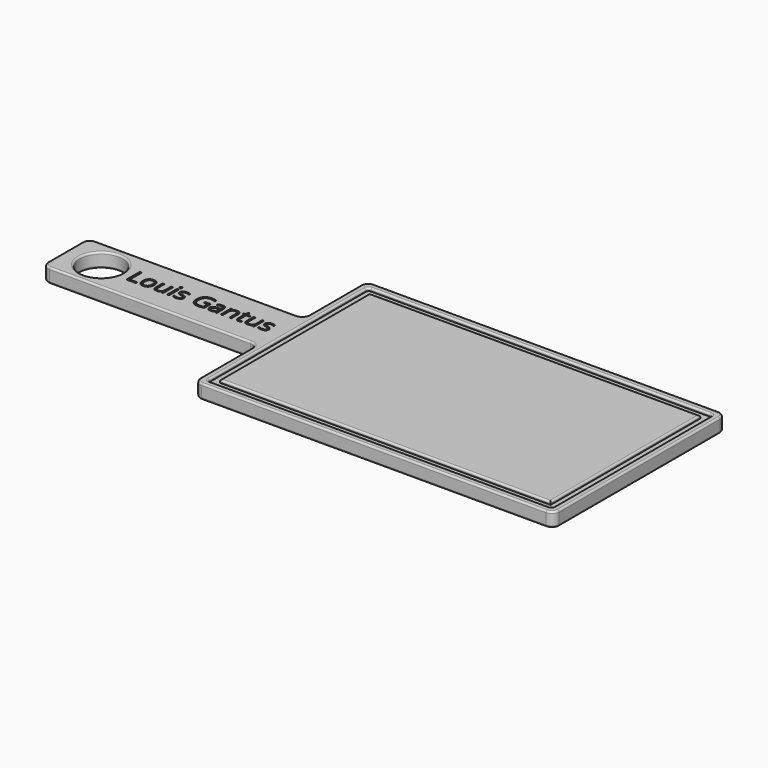
from build123d import *

# Parameters (mm, degrees)
F0_W         = 381
F0_H         = 101.6
F1_DEPTH     = 25.4
F2_R         = 38.1
F3_DEPTH     = 25.4
F5_DEPTH     = 5.08
F6_R         = 5.08
F7_R         = 12.7
F8_R         = 3.175
F9_TEXT_SIZE = 41.7269880384
F10_DEPTH    = 3.175


# Not quite as in the source:
# - Text() gives the source's letters only with a copy of the font that has no kerning and outlines rounded to 1/6400 em; it was checked with that copy


with BuildPart() as f1:
    # F0 (on Top) → F1 (new body)
    with BuildSketch(Plane.XY):
        Polygon((0, 139.7), (0, 0), (635, 0), (635, 381), (0, 381), (0, 241.3), align=None)
        with Locations((-190.5, 190.5)):
            Rectangle(F0_W, F0_H)
    extrude(amount=F1_DEPTH)

    # F2 (on face) → F3 (cut)
    with BuildSketch(Plane.XY.offset(25.4)):
        with Locations((-317.5, 190.5)):
            Circle(F2_R)
    extrude(amount=-F3_DEPTH, mode=Mode.SUBTRACT)

    # F4 (on face) → F5 (cut)
    with BuildSketch(Plane.XY.offset(25.4)):
        Polygon((12.4460039139, 139.7), (12.4460039139, 12.4460039139), (622.5539960861, 12.4460039139), (622.5539960861, 368.5539960861), (12.4460039139, 368.5539960861), (12.4460039139, 241.3), align=None)
        Polygon((24.8919901848, 139.7), (24.8919901848, 241.3), (24.8919901848, 356.1080098152), (610.1080098152, 356.1080098152), (610.1080098152, 24.8919901848), (24.8919901848, 24.8919901848), align=None, mode=Mode.SUBTRACT)
    extrude(amount=-F5_DEPTH, mode=Mode.SUBTRACT)

    # F6
    f6_edges = [f1.edges().sort_by_distance(p)[0] for p in [
        (12.446004, 368.553996, 22.86),
        (622.553996, 368.553996, 22.86),
        (12.446004, 12.446004, 22.86),
        (622.553996, 12.446004, 22.86),
    ]]
    fillet(f6_edges, radius=F6_R)

    # F7
    f7_edges = [f1.edges().sort_by_distance(p)[0] for p in [
        (0, 0, 12.7),
        (0, 139.7, 12.7),
        (-381, 139.7, 12.7),
        (-381, 241.3, 12.7),
        (0, 241.3, 12.7),
        (0, 381, 12.7),
        (635, 0, 12.7),
        (635, 381, 12.7),
    ]]
    fillet(f7_edges, radius=F7_R)

    # F8
    f8_edges = [f1.edges().sort_by_distance(p)[0] for p in [
        (317.5, 356.10801, 25.4),
        (610.10801, 190.5, 25.4),
        (317.5, 24.89199, 25.4),
        (24.89199, 190.5, 25.4),
        (0, 69.85, 25.4),
        (-3.719744, 135.980256, 25.4),
        (3.719744, 3.719744, 25.4),
        (-190.5, 139.7, 25.4),
        (317.5, 0, 25.4),
        (-377.280256, 143.419744, 25.4),
        (631.280256, 3.719744, 25.4),
        (-381, 190.5, 25.4),
        (635, 190.5, 25.4),
        (-377.280256, 237.580256, 25.4),
        (631.280256, 377.280256, 25.4),
        (-190.5, 241.3, 25.4),
        (317.5, 381, 25.4),
        (-3.719744, 245.019744, 25.4),
        (3.719744, 377.280256, 25.4),
        (0, 311.15, 25.4),
        (317.5, 12.446004, 25.4),
        (13.933901, 13.933901, 25.4),
        (621.066099, 13.933901, 25.4),
        (12.446004, 190.5, 25.4),
        (622.553996, 190.5, 25.4),
        (13.933901, 367.066099, 25.4),
        (621.066099, 367.066099, 25.4),
        (317.5, 368.553996, 25.4),
        (-355.6, 190.5, 25.4),
        (0, 69.85, 0),
        (-3.719744, 135.980256, 0),
        (3.719744, 3.719744, 0),
        (-190.5, 139.7, 0),
        (317.5, 0, 0),
        (-377.280256, 143.419744, 0),
        (631.280256, 3.719744, 0),
        (-381, 190.5, 0),
        (635, 190.5, 0),
        (-377.280256, 237.580256, 0),
        (631.280256, 377.280256, 0),
        (-190.5, 241.3, 0),
        (317.5, 381, 0),
        (-3.719744, 245.019744, 0),
        (3.719744, 377.280256, 0),
        (0, 311.15, 0),
        (-355.6, 190.5, 0),
    ]]
    fillet(f8_edges, radius=F8_R)

    # F9 (on face) → F10 (cut)
    with BuildSketch(Plane.XY.offset(25.4)):
        with Locations((-266.7601889959, 177.7769717114)):
            Text('Louis Gantus', F9_TEXT_SIZE, font='Open Sans', text_align=(TextAlign.LEFT, TextAlign.BOTTOM))
    extrude(amount=-F10_DEPTH, mode=Mode.SUBTRACT)


solid = f1.part
